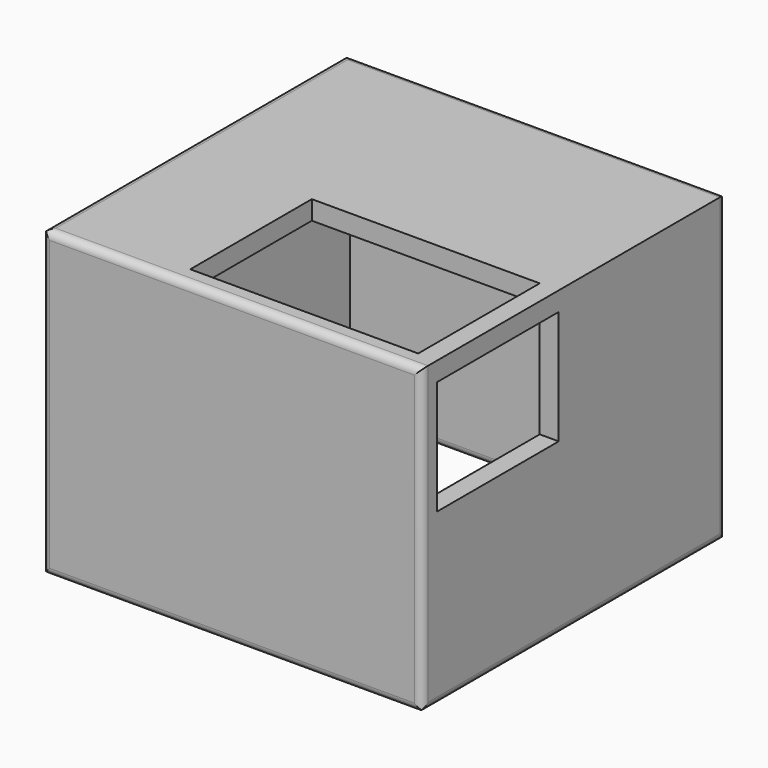
from build123d import *

# Parameters (mm, degrees)
F0_W          = 254
F0_H          = 254
F0_W_2        = 228.6
F0_H_2        = 228.6
F1_DEPTH      = 203.2
F2_T          = -12.7
F3_W          = 152.4
F3_H          = 101.6
F4_DEPTH      = 12.7
F5_W          = 101.6
F5_H          = 76.2
F6_DEPTH      = 76.2
F7_R          = 5.08
F8_R          = 5.08
F9_T1_DEPTH   = 269.24
F10_T1_DEPTH  = 269.24
F10_T3_DEPTH  = 228.6
F10_T5_DEPTH  = 228.6
F10_T11_DEPTH = 241.3
F10_T15_DEPTH = 241.3
F10_T22_DEPTH = 241.3
F10_T26_DEPTH = 241.3
F10_T33_DEPTH = 241.3
F10_T37_DEPTH = 241.3
F10_T44_DEPTH = 241.3
F10_T48_DEPTH = 241.3


# Not quite as in the source:
# - a fillet or chamfer that OpenCascade refuses, or shapes differently, is made with other operations: its cross-section is extruded or revolved along the edge and cut away or added


with BuildPart() as f1:
    # F0 (on Top) → F1 (new body)
    with BuildSketch(Plane.XY):
        with Locations((-74.773899883, 78.5929929912)):
            Rectangle(F0_W, F0_H)
        with Locations((-74.773899883, 78.5929929912)):
            Rectangle(F0_W_2, F0_H_2, mode=Mode.SUBTRACT)
        with Locations((-74.773899883, 78.5929929912)):
            Rectangle(F0_W_2, F0_H_2)
    extrude(amount=-F1_DEPTH)

    # F2
    f2_openings = [f1.faces().sort_by_distance(p)[0] for p in [
        (-74.7739, 78.592993, -203.2),
    ]]
    offset(amount=F2_T, openings=f2_openings)

    # F3 (on Top) → F4 (cut)
    with BuildSketch(Plane.XY):
        with Locations((-36.673899883, 15.0929929912)):
            Rectangle(F3_W, F3_H)
    extrude(amount=-F4_DEPTH, mode=Mode.SUBTRACT)

    # F5 (on Right) → F6 (cut)
    with BuildSketch(Plane.YZ):
        with Locations((15.0929929912, -50.8)):
            Rectangle(F5_W, F5_H)
    extrude(amount=F6_DEPTH, mode=Mode.SUBTRACT)

    # F7
    f7_edges = [f1.edges().sort_by_distance(p)[0] for p in [
        (52.2261, 205.592993, -101.6),
        (-201.7739, 205.592993, -101.6),
        (-74.7739, 205.592993, 0),
        (-74.7739, 205.592993, -203.2),
    ]]
    fillet(f7_edges, radius=F7_R)

    # F8
    f8_edges = [f1.edges().sort_by_distance(p)[0] for p in [
        (-201.7739, -48.407007, -101.6),
        (52.2261, -48.407007, -101.6),
        (-74.7739, -48.407007, 0),
        (-74.7739, -48.407007, -203.2),
    ]]
    fillet(f8_edges, radius=F8_R)

    # F9: fillet of radius 5.08 on 4 edges, made by hand

    # F9_s2 → F9_t1 (cut)
    with BuildSketch(Plane.XZ.offset(-213.2129929912)):
        with BuildLine():
            ThreePointArc((-196.693899883, 0), (-200.2860023315, -1.4878975516), (-201.773899883, -5.08))
            Line((-201.773899883, -5.08), (-201.773899883, 0))
            Line((-201.773899883, 0), (-196.693899883, 0))
        make_face()
        with BuildLine():
            ThreePointArc((-196.693899883, -203.2), (-200.2860023315, -201.7121024484), (-201.773899883, -198.12))
            Line((-201.773899883, -198.12), (-201.773899883, -203.2))
            Line((-201.773899883, -203.2), (-196.693899883, -203.2))
        make_face()
    extrude(amount=F9_T1_DEPTH, mode=Mode.SUBTRACT)

    # F10: fillet of radius 5.08 on 8 edges, made by hand

    # F10_s2 → F10_t1 (cut)
    with BuildSketch(Plane.XZ.offset(-213.2129929912)):
        with BuildLine():
            ThreePointArc((52.226100117, -198.12), (50.7382025654, -201.7121024484), (47.146100117, -203.2))
            Line((47.146100117, -203.2), (52.226100117, -203.2))
            Line((52.226100117, -203.2), (52.226100117, -198.12))
        make_face()
    extrude(amount=F10_T1_DEPTH, mode=Mode.SUBTRACT)

    # F10_s4 → F10_t3 (cut)
    with BuildSketch(Plane.XZ.offset(-192.8929929912)):
        with BuildLine():
            ThreePointArc((44.606100117, -203.2), (41.0139976685, -201.7121024484), (39.526100117, -198.12))
            Line((39.526100117, -198.12), (39.526100117, -203.2))
            Line((39.526100117, -203.2), (44.606100117, -203.2))
        make_face()
        with BuildLine():
            ThreePointArc((-194.153899883, -203.2), (-190.5617974346, -201.7121024484), (-189.073899883, -198.12))
            Line((-189.073899883, -198.12), (-189.073899883, -203.2))
            Line((-189.073899883, -203.2), (-194.153899883, -203.2))
        make_face()
    extrude(amount=F10_T3_DEPTH, mode=Mode.SUBTRACT)

    # F10_s6 → F10_t5 (cut)
    with BuildSketch(Plane.YZ.offset(-189.073899883)):
        with BuildLine():
            ThreePointArc((-40.7870070088, -203.2), (-37.1949045604, -201.7121024484), (-35.7070070088, -198.12))
            Line((-35.7070070088, -198.12), (-35.7070070088, -203.2))
            Line((-35.7070070088, -203.2), (-40.7870070088, -203.2))
        make_face()
        with BuildLine():
            ThreePointArc((197.9729929912, -203.2), (194.3808905428, -201.7121024484), (192.8929929912, -198.12))
            Line((192.8929929912, -198.12), (192.8929929912, -203.2))
            Line((192.8929929912, -203.2), (197.9729929912, -203.2))
        make_face()
    extrude(amount=F10_T5_DEPTH, mode=Mode.SUBTRACT)


with BuildPart() as f10_tool9:
    # F10_s10 → F10_t11 (new body)
    with BuildSketch(Plane.XZ.offset(48.4070070088)):
        with BuildLine():
            ThreePointArc((44.606100117, -203.2), (41.0139976685, -201.7121024484), (39.526100117, -198.12))
            Line((39.526100117, -198.12), (39.526100117, -203.2))
            Line((39.526100117, -203.2), (44.606100117, -203.2))
        make_face()
    extrude(amount=-F10_T11_DEPTH)

    split(bisect_by=Plane.XZ.offset(35.7070070088), keep=Keep.TOP)


with BuildPart() as f10_tool13:
    # F10_s14 → F10_t15 (new body)
    with BuildSketch(Plane.YZ.offset(-189.073899883)):
        with BuildLine():
            ThreePointArc((-40.7870070088, -203.2), (-37.1949045604, -201.7121024484), (-35.7070070088, -198.12))
            Line((-35.7070070088, -198.12), (-35.7070070088, -203.2))
            Line((-35.7070070088, -203.2), (-40.7870070088, -203.2))
        make_face()
    extrude(amount=F10_T15_DEPTH)

    split(bisect_by=Plane.YZ.offset(39.526100117), keep=Keep.TOP)


with BuildPart() as f10_tool9_1:
    add(f10_tool9.part)

    # F10_t17: intersect F10_tool13
    add(f10_tool13.part, mode=Mode.INTERSECT)


with BuildPart() as f1_1:
    add(f1.part)

    # F10_t7: cut F10_tool9
    add(f10_tool9_1.part, mode=Mode.SUBTRACT)


with BuildPart() as f10_tool20:
    # F10_s21 → F10_t22 (new body)
    with BuildSketch(Plane.XZ.offset(35.7070070088)):
        with BuildLine():
            ThreePointArc((44.606100117, -203.2), (41.0139976685, -201.7121024484), (39.526100117, -198.12))
            Line((39.526100117, -198.12), (39.526100117, -203.2))
            Line((39.526100117, -203.2), (44.606100117, -203.2))
        make_face()
    extrude(amount=-F10_T22_DEPTH)

    split(bisect_by=Plane.XZ.offset(-192.8929929912), keep=Keep.BOTTOM)


with BuildPart() as f10_tool24:
    # F10_s25 → F10_t26 (new body)
    with BuildSketch(Plane.YZ.offset(52.226100117)):
        with BuildLine():
            ThreePointArc((197.9729929912, -203.2), (194.3808905428, -201.7121024484), (192.8929929912, -198.12))
            Line((192.8929929912, -198.12), (192.8929929912, -203.2))
            Line((192.8929929912, -203.2), (197.9729929912, -203.2))
        make_face()
    extrude(amount=-F10_T26_DEPTH)

    split(bisect_by=Plane.YZ.offset(39.526100117), keep=Keep.TOP)


with BuildPart() as f10_tool20_1:
    add(f10_tool20.part)

    # F10_t28: intersect F10_tool24
    add(f10_tool24.part, mode=Mode.INTERSECT)


with BuildPart() as f1_2:
    add(f1_1.part)

    # F10_t18: cut F10_tool20
    add(f10_tool20_1.part, mode=Mode.SUBTRACT)


with BuildPart() as f10_tool31:
    # F10_s32 → F10_t33 (new body)
    with BuildSketch(Plane.YZ.offset(-201.773899883)):
        with BuildLine():
            ThreePointArc((-40.7870070088, -203.2), (-37.1949045604, -201.7121024484), (-35.7070070088, -198.12))
            Line((-35.7070070088, -198.12), (-35.7070070088, -203.2))
            Line((-35.7070070088, -203.2), (-40.7870070088, -203.2))
        make_face()
    extrude(amount=F10_T33_DEPTH)

    split(bisect_by=Plane.YZ.offset(-189.073899883), keep=Keep.BOTTOM)


with BuildPart() as f10_tool35:
    # F10_s36 → F10_t37 (new body)
    with BuildSketch(Plane.XZ.offset(-192.8929929912)):
        with BuildLine():
            ThreePointArc((-194.153899883, -203.2), (-190.5617974346, -201.7121024484), (-189.073899883, -198.12))
            Line((-189.073899883, -198.12), (-189.073899883, -203.2))
            Line((-189.073899883, -203.2), (-194.153899883, -203.2))
        make_face()
    extrude(amount=F10_T37_DEPTH)

    split(bisect_by=Plane.XZ.offset(35.7070070088), keep=Keep.TOP)


with BuildPart() as f10_tool31_1:
    add(f10_tool31.part)

    # F10_t39: intersect F10_tool35
    add(f10_tool35.part, mode=Mode.INTERSECT)


with BuildPart() as f1_3:
    add(f1_2.part)

    # F10_t29: cut F10_tool31
    add(f10_tool31_1.part, mode=Mode.SUBTRACT)


with BuildPart() as f10_tool42:
    # F10_s43 → F10_t44 (new body)
    with BuildSketch(Plane.YZ.offset(39.526100117)):
        with BuildLine():
            ThreePointArc((197.9729929912, -203.2), (194.3808905428, -201.7121024484), (192.8929929912, -198.12))
            Line((192.8929929912, -198.12), (192.8929929912, -203.2))
            Line((192.8929929912, -203.2), (197.9729929912, -203.2))
        make_face()
    extrude(amount=-F10_T44_DEPTH)

    split(bisect_by=Plane.YZ.offset(-189.073899883), keep=Keep.BOTTOM)


with BuildPart() as f10_tool46:
    # F10_s47 → F10_t48 (new body)
    with BuildSketch(Plane.XZ.offset(-205.5929929912)):
        with BuildLine():
            ThreePointArc((-194.153899883, -203.2), (-190.5617974346, -201.7121024484), (-189.073899883, -198.12))
            Line((-189.073899883, -198.12), (-189.073899883, -203.2))
            Line((-189.073899883, -203.2), (-194.153899883, -203.2))
        make_face()
    extrude(amount=F10_T48_DEPTH)

    split(bisect_by=Plane.XZ.offset(-192.8929929912), keep=Keep.BOTTOM)


with BuildPart() as f10_tool42_1:
    add(f10_tool42.part)

    # F10_t50: intersect F10_tool46
    add(f10_tool46.part, mode=Mode.INTERSECT)


with BuildPart() as f1_4:
    add(f1_3.part)

    # F10_t40: cut F10_tool42
    add(f10_tool42_1.part, mode=Mode.SUBTRACT)


solid = f1_4.part
